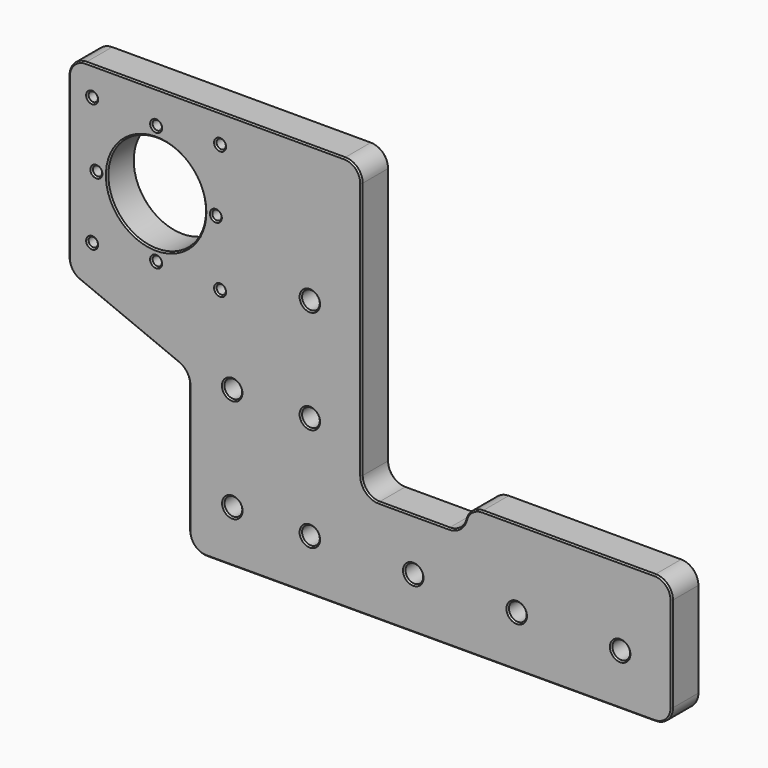
from build123d import *

# Parameters (mm, degrees)
F0_R     = 3.2639
F0_R_2   = 1.7018
F0_R_3   = 17.9959
F1_DEPTH = 12.7
F2_W     = 107.95
F2_H     = 19.1731796932
F3_DEPTH = 25.4
F4_F1_R  = 6.35
F4_F2_R  = 6.35
F5_R     = 6.35
F6_SIZE  = 0.508


# Not quite as in the source:
# - a feature names something its author has since deleted; it is built from what else it names


with BuildPart() as f1:
    # F0 (on Front) → F1 (new body)
    with BuildSketch(Plane.XZ):
        Polygon((-126.667948618, -98.8461842824), (95.582051382, -98.5286048876), (95.582051382, -60.4286048876), (95.582051382, -50.9036048876), (19.382051382, -50.9036048876), (19.382051382, -60.4286048876), (-18.717948618, -60.4286048876), (-18.717948618, 66.2538157176), (-126.667948618, 66.2538157176), align=None)
        with Locations((-66.3308787224, -79.5945032566)):
            Circle(F0_R, mode=Mode.SUBTRACT)
        with Locations((-37.7828981478, -79.6691544378)):
            Circle(F0_R, mode=Mode.SUBTRACT)
        with Locations((-66.3853614397, -41.4661356021)):
            Circle(F0_R, mode=Mode.SUBTRACT)
        with Locations((-37.7829381848, -41.4661356021)):
            Circle(F0_R, mode=Mode.SUBTRACT)
        with Locations((0.3171018521, -79.6691544378)):
            Circle(F0_R, mode=Mode.SUBTRACT)
        with Locations((38.4171018521, -79.6691544378)):
            Circle(F0_R, mode=Mode.SUBTRACT)
        with Locations((76.5171018521, -79.6691544378)):
            Circle(F0_R, mode=Mode.SUBTRACT)
        with Locations((-117.9733242227, -10.6661073038)):
            Circle(F0_R_2, mode=Mode.SUBTRACT)
        with Locations((-94.4033242227, -9.0925073038)):
            Circle(F0_R_2, mode=Mode.SUBTRACT)
        with Locations((-116.3997242227, 12.9038926962)):
            Circle(F0_R_2, mode=Mode.SUBTRACT)
        with Locations((-94.4033242227, 12.9038926962)):
            Circle(F0_R_3, mode=Mode.SUBTRACT)
        with Locations((-72.4069242227, 12.9038926962)):
            Circle(F0_R_2, mode=Mode.SUBTRACT)
        with Locations((-70.8333242227, -10.6661073038)):
            Circle(F0_R_2, mode=Mode.SUBTRACT)
        with Locations((-37.7829381848, -3.3661356021)):
            Circle(F0_R, mode=Mode.SUBTRACT)
        with Locations((-117.9733242227, 36.4738926962)):
            Circle(F0_R_2, mode=Mode.SUBTRACT)
        with Locations((-94.4033242227, 34.9002926962)):
            Circle(F0_R_2, mode=Mode.SUBTRACT)
        with Locations((-70.8333242227, 36.4738926962)):
            Circle(F0_R_2, mode=Mode.SUBTRACT)
    extrude(amount=F1_DEPTH)

    # F2 (on face) → F3 (cut)
    with BuildSketch(Plane.XZ.offset(12.7)):
        Polygon((-82.2600983048, -40.9187248283), (-126.667948618, -22.6552803069), (-126.667948618, -98.8461842824), (-82.2600983048, -98.7827286323), align=None)
        with Locations((-72.692948618, 56.6672258711)):
            Rectangle(F2_W, F2_H)
    extrude(amount=-F3_DEPTH, mode=Mode.SUBTRACT)

    # F4: fillet of radius 6.35 on 9 edges, made by hand

    # F4_f1
    f4_f1_edges = [f1.edges().sort_by_distance(p)[0] for p in [
        (-82.2600983048, -6.35, -40.9187248283),
        (-18.717948618, -6.35, -60.4286048876),
    ]]
    fillet(f4_f1_edges, radius=F4_F1_R)

    # F4_f2
    f4_f2_edges = [f1.edges().sort_by_distance(p)[0] for p in [
        (-126.667948618, -6.35, 47.0806360245),
        (-126.667948618, -6.35, -22.6552803069),
        (-18.717948618, -6.35, 47.0806360245),
        (-82.2600983048, -6.35, -98.7827286323),
        (95.582051382, -6.35, -98.5286048876),
        (95.582051382, -6.35, -50.9036048876),
        (19.382051382, -6.35, -50.9036048876),
    ]]
    fillet(f4_f2_edges, radius=F4_F2_R)

    # F5
    f5_edges = [f1.edges().sort_by_distance(p)[0] for p in [
        (19.382051, -6.35, -60.428605),
    ]]
    fillet(f5_edges, radius=F5_R)

    # F6
    f6_edges = [f1.edges().sort_by_distance(p)[0] for p in [
        (21.843486, -12.7, -52.233489),
        (17.323894, -12.7, -59.098721),
        (57.482051, -12.7, -50.903605),
        (0.53369, -12.7, -60.428605),
        (93.722179, -12.7, -52.763477),
        (-16.858077, -12.7, -58.568733),
        (95.582051, -12.7, -74.720638),
        (-18.717949, -12.7, -6.673984),
        (93.725386, -12.7, -96.674591),
        (-20.577821, -12.7, 45.220764),
        (6.67005, -12.7, -98.655654),
        (-72.692949, -12.7, 47.080636),
        (-80.397017, -12.7, -96.916983),
        (-124.808077, -12.7, 45.220764),
        (-82.260098, -12.7, -68.798442),
        (-126.667949, -12.7, 11.164933),
        (-83.334713, -12.7, -41.638718),
        (-125.593334, -12.7, -21.935287),
        (-104.464023, -12.7, -31.787003),
        (-69.594779, -12.7, -79.594503),
        (-41.046798, -12.7, -79.669154),
        (-69.649261, -12.7, -41.466136),
        (-41.046838, -12.7, -41.466136),
        (-2.946798, -12.7, -79.669154),
        (35.153202, -12.7, -79.669154),
        (73.253202, -12.7, -79.669154),
        (-119.675124, -12.7, -10.666107),
        (-96.105124, -12.7, -9.092507),
        (-72.535124, -12.7, -10.666107),
        (-41.046838, -12.7, -3.366136),
        (-118.101524, -12.7, 12.903893),
        (-112.399224, -12.7, 12.903893),
        (-74.108724, -12.7, 12.903893),
        (-119.675124, -12.7, 36.473893),
        (-96.105124, -12.7, 34.900293),
        (-72.535124, -12.7, 36.473893),
        (21.843486, 0, -52.233489),
        (17.323894, 0, -59.098721),
        (57.482051, 0, -50.903605),
        (0.53369, 0, -60.428605),
        (93.722179, 0, -52.763477),
        (-16.858077, 0, -58.568733),
        (95.582051, 0, -74.720638),
        (-18.717949, 0, -6.673984),
        (93.725386, 0, -96.674591),
        (-20.577821, 0, 45.220764),
        (6.67005, 0, -98.655654),
        (-72.692949, 0, 47.080636),
        (-80.397017, 0, -96.916983),
        (-124.808077, 0, 45.220764),
        (-82.260098, 0, -68.798442),
        (-126.667949, 0, 11.164933),
        (-83.334713, 0, -41.638718),
        (-125.593334, 0, -21.935287),
        (-104.464023, 0, -31.787003),
        (-69.594779, 0, -79.594503),
        (-41.046798, 0, -79.669154),
        (-69.649261, 0, -41.466136),
        (-41.046838, 0, -41.466136),
        (-2.946798, 0, -79.669154),
        (35.153202, 0, -79.669154),
        (73.253202, 0, -79.669154),
        (-119.675124, 0, -10.666107),
        (-96.105124, 0, -9.092507),
        (-72.535124, 0, -10.666107),
        (-41.046838, 0, -3.366136),
        (-118.101524, 0, 12.903893),
        (-112.399224, 0, 12.903893),
        (-74.108724, 0, 12.903893),
        (-119.675124, 0, 36.473893),
        (-96.105124, 0, 34.900293),
        (-72.535124, 0, 36.473893),
    ]]
    chamfer(f6_edges, length=F6_SIZE)


solid = f1.part
